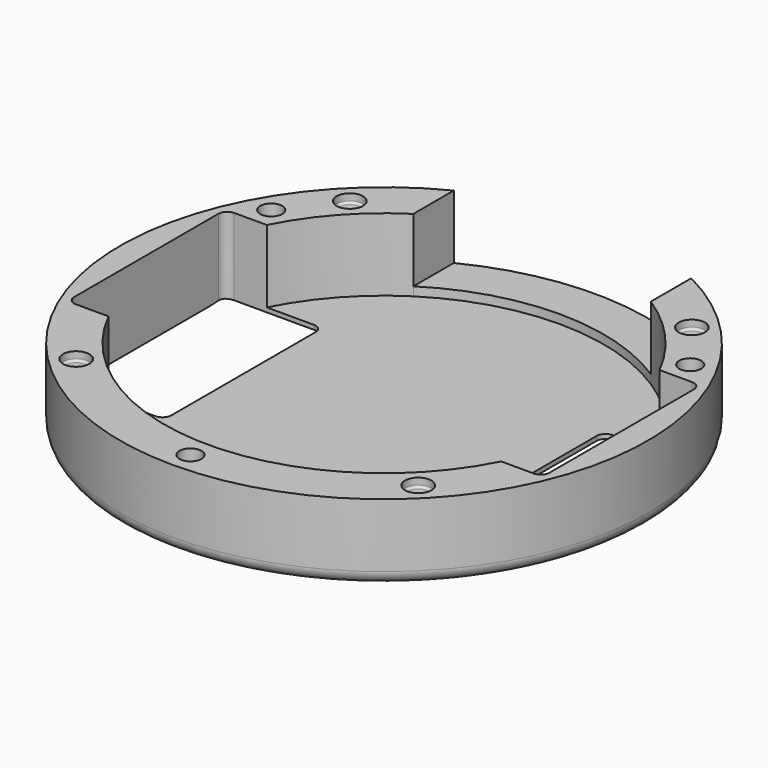
from build123d import *

# Parameters (mm, degrees)
F1_DEPTH  = 17.5
F2_R      = 3
F3_DEPTH  = 2
F2_R_2    = 2.5
F4_DEPTH  = 5
F5_R      = 0.5
F6_R      = 1.5
F10_DEPTH = 1
F11_DEPTH = 3
F13_R     = 2


# Not quite as in the source:
# - a fillet or chamfer that OpenCascade refuses, or shapes differently, is made with other operations: its cross-section is extruded or revolved along the edge and cut away or added
# - a feature names something its author has since deleted; it is built from what else it names


with BuildPart() as f1:
    # F0 (on Top) → F1 (new body)
    with BuildSketch(Plane.XY):
        with BuildLine():
            ThreePointArc((-27, 53.5817132985), (-31.4642654451, -51.0881590978), (60, 0))
            ThreePointArc((60, 0), (51.0881590978, 31.4642654451), (27, 53.5817132985))
            Line((27, 53.5817132985), (27, 42.083250825))
            ThreePointArc((27, 42.083250825), (37.1397052065, 33.4759958354), (44.6514277487, 22.5))
            Line((44.6514277487, 22.5), (54.0514277487, 22.5))
            Line((54.0514277487, 22.5), (54.0514277487, -22.5))
            Line((54.0514277487, -22.5), (44.6514277487, -22.5))
            ThreePointArc((44.6514277487, -22.5), (0, -50), (-44.6514277487, -22.5))
            Line((-44.6514277487, -22.5), (-54.0514277487, -22.5))
            Line((-54.0514277487, -22.5), (-54.0514277487, 22.5))
            Line((-54.0514277487, 22.5), (-44.6514277487, 22.5))
            ThreePointArc((-44.6514277487, 22.5), (-37.1397052065, 33.4759958354), (-27, 42.083250825))
            Line((-27, 42.083250825), (-27, 53.5817132985))
        make_face()
    extrude(amount=F1_DEPTH)

    # F2 (on face) → F3 (cut)
    with BuildSketch(Plane.XY.offset(17.5)):
        with Locations((-38.8908729653, 38.8908729653)):
            Circle(F2_R)
        with Locations((38.8908729653, 38.8908729653)):
            Circle(F2_R)
        with Locations((38.8908729653, -38.8908729653)):
            Circle(F2_R)
        with Locations((-38.8908729653, -38.8908729653)):
            Circle(F2_R)
    extrude(amount=-F3_DEPTH, mode=Mode.SUBTRACT)

    # F2 (on face) → F4 (cut)
    with BuildSketch(Plane.XY.offset(17.5)):
        with Locations((0, -55)):
            Circle(F2_R_2)
        with Locations((47.6313972081, 27.5)):
            Circle(F2_R_2)
        with Locations((-47.6313972081, 27.5)):
            Circle(F2_R_2)
    extrude(amount=-F4_DEPTH, mode=Mode.SUBTRACT)

    # F5
    f5_edges = [f1.edges().sort_by_distance(p)[0] for p in [
        (35.890873, -38.890873, 15.5),
        (-41.890873, -38.890873, 15.5),
        (-41.890873, 38.890873, 15.5),
        (35.890873, 38.890873, 15.5),
    ]]
    fillet(f5_edges, radius=F5_R)

    # F6
    f6_edges = [f1.edges().sort_by_distance(p)[0] for p in [
        (-2.5, -55, 12.5),
        (45.131397, 27.5, 12.5),
        (-50.131397, 27.5, 12.5),
    ]]
    fillet(f6_edges, radius=F6_R)


with BuildPart() as f7_1:
    # F7: copy of F1
    add(f1.part)


with BuildPart() as f1_1:
    add(f1.part)

    # F0 (on Top) → F10 (join)
    with BuildSketch(Plane.XY):
        with BuildLine():
            ThreePointArc((44.6514277487, 22.5), (37.1397052065, 33.4759958354), (27, 42.083250825))
            ThreePointArc((27, 42.083250825), (0, 50), (-27, 42.083250825))
            ThreePointArc((-27, 42.083250825), (-37.1397052065, 33.4759958354), (-44.6514277487, 22.5))
            Line((-44.6514277487, 22.5), (-31.9514277487, 22.5))
            Line((-31.9514277487, 22.5), (-31.9514277487, -22.5))
            Line((-31.9514277487, -22.5), (-44.6514277487, -22.5))
            ThreePointArc((-44.6514277487, -22.5), (0, -50), (44.6514277487, -22.5))
            Line((44.6514277487, -22.5), (31.9514277487, -22.5))
            Line((31.9514277487, -22.5), (31.9514277487, 22.5))
            Line((31.9514277487, 22.5), (44.6514277487, 22.5))
        make_face()
        with BuildLine():
            Line((-30.3973683071, -26), (30.3973683071, -26))
            ThreePointArc((30.3973683071, -26), (0, -40), (-30.3973683071, -26))
        make_face(mode=Mode.SUBTRACT)
    extrude(amount=F10_DEPTH)

    # F0 (on Top) → F11 (join)
    with BuildSketch(Plane.XY):
        with BuildLine():
            Line((27, 42.083250825), (27, 53.5817132985))
            ThreePointArc((27, 53.5817132985), (0, 60), (-27, 53.5817132985))
            Line((-27, 53.5817132985), (-27, 42.083250825))
            ThreePointArc((-27, 42.083250825), (0, 50), (27, 42.083250825))
        make_face()
    extrude(amount=F11_DEPTH)

    # F12: fillet of radius 3 on 1 edges, made by hand

    # F12_s1 → F12_t2 (revolve, cut)
    with BuildSketch(Plane.XZ):
        with BuildLine():
            ThreePointArc((57, 0), (59.1213203436, 0.8786796564), (60, 3))
            Line((60, 3), (60, 0))
            Line((60, 0), (57, 0))
        make_face()
    revolve(axis=Axis((0, 0, 0), (0, 0, 1)), mode=Mode.SUBTRACT)

    # F13#2 (call 1 of 8: OpenCascade refuses the feature's edges together)
    f13_2_edges = [f1_1.edges().sort_by_distance(p)[0] for p in [
        (31.951428, 22.5, 0.5),
    ]]
    fillet(f13_2_edges, radius=F13_R)

    # F13#3 (call 2 of 8)
    f13_3_edges = [f1_1.edges().sort_by_distance(p)[0] for p in [
        (31.951428, -22.5, 0.5),
    ]]
    fillet(f13_3_edges, radius=F13_R)

    # F13#4 (call 3 of 8)
    f13_4_edges = [f1_1.edges().sort_by_distance(p)[0] for p in [
        (54.051428, -22.5, 8.964959),
    ]]
    fillet(f13_4_edges, radius=F13_R)

    # F13#6 (call 4 of 8)
    f13_6_edges = [f1_1.edges().sort_by_distance(p)[0] for p in [
        (-54.051428, -22.5, 8.964959),
    ]]
    fillet(f13_6_edges, radius=F13_R)

    # F13#7 (call 5 of 8)
    f13_7_edges = [f1_1.edges().sort_by_distance(p)[0] for p in [
        (-31.951428, 22.5, 0.5),
    ]]
    fillet(f13_7_edges, radius=F13_R)

    # F13#8 (call 6 of 8)
    f13_8_edges = [f1_1.edges().sort_by_distance(p)[0] for p in [
        (-31.951428, -22.5, 0.5),
    ]]
    fillet(f13_8_edges, radius=F13_R)

    # F13 (call 7 of 8)
    f13_edges = [f1_1.edges().sort_by_distance(p)[0] for p in [
        (54.051428, 22.5, 8.964959),
    ]]
    fillet(f13_edges, radius=F13_R)

    # F13#5 (call 8 of 8)
    f13_5_edges = [f1_1.edges().sort_by_distance(p)[0] for p in [
        (-54.051428, 22.5, 8.964959),
    ]]
    fillet(f13_5_edges, radius=F13_R)


solid = f1_1.part
